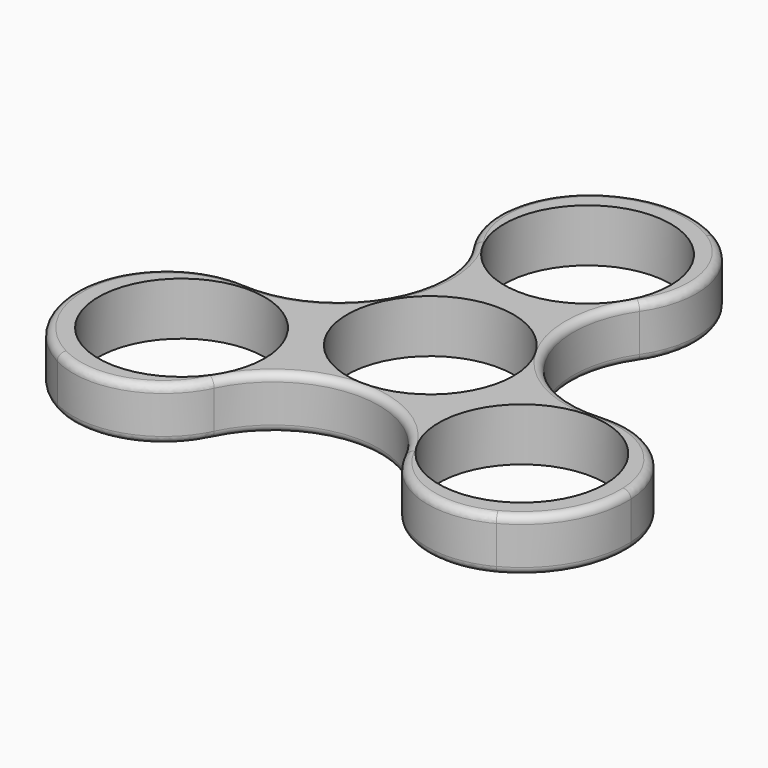
from build123d import *

# Parameters (mm, degrees)
F0_R     = 11
F1_DEPTH = 7
F2_R     = 12
F3_R     = 0.99999
F4_R     = 0.99999


# Not quite as in the source:
# - a fillet or chamfer is up to 0.001 mm smaller than in the source, because OpenCascade refuses the exact size


with BuildPart() as f1:
    # F0 (on Top) → F1 (new body)
    with BuildSketch(Plane.XY):
        with BuildLine():
            ThreePointArc((27.7128129211, 0), (10.3923048454, 6), (13.8564064606, 24))
            ThreePointArc((13.8564064606, 24), (0, 40), (-13.8564064606, 24))
            ThreePointArc((-13.8564064606, 24), (-10.3923048454, 6), (-27.7128129211, 0))
            ThreePointArc((-27.7128129211, 0), (-34.6410161514, -20), (-13.8564064606, -24))
            ThreePointArc((-13.8564064606, -24), (0, -12), (13.8564064606, -24))
            ThreePointArc((13.8564064606, -24), (34.6410161514, -20), (27.7128129211, 0))
        make_face()
        with Locations((-22.5166604984, -13)):
            Circle(F0_R, mode=Mode.SUBTRACT)
        with Locations((22.5166604984, -13)):
            Circle(F0_R, mode=Mode.SUBTRACT)
        Circle(F0_R, mode=Mode.SUBTRACT)
        with Locations((0, 26)):
            Circle(F0_R, mode=Mode.SUBTRACT)
    extrude(amount=F1_DEPTH)

    # F2
    f2_edges = [f1.edges().sort_by_distance(p)[0] for p in [
        (-13.856406, 24, 3.5),
        (-27.712813, 0, 3.5),
        (27.712813, 0, 3.5),
        (13.856406, -24, 3.5),
        (13.856406, 24, 3.5),
        (-13.856406, -24, 3.5),
    ]]
    fillet(f2_edges, radius=F2_R)

    # F3 (radius 1 in the source; OpenCascade refuses exactly that, so slightly less here)
    f3_edges = [f1.edges().sort_by_distance(p)[0] for p in [
        (0, -12, 0),
    ]]
    fillet(f3_edges, radius=F3_R)

    # F4 (radius 1 in the source; OpenCascade refuses exactly that, so slightly less here)
    f4_edges = [f1.edges().sort_by_distance(p)[0] for p in [
        (10.392305, 6, 7),
    ]]
    fillet(f4_edges, radius=F4_R)


solid = f1.part
